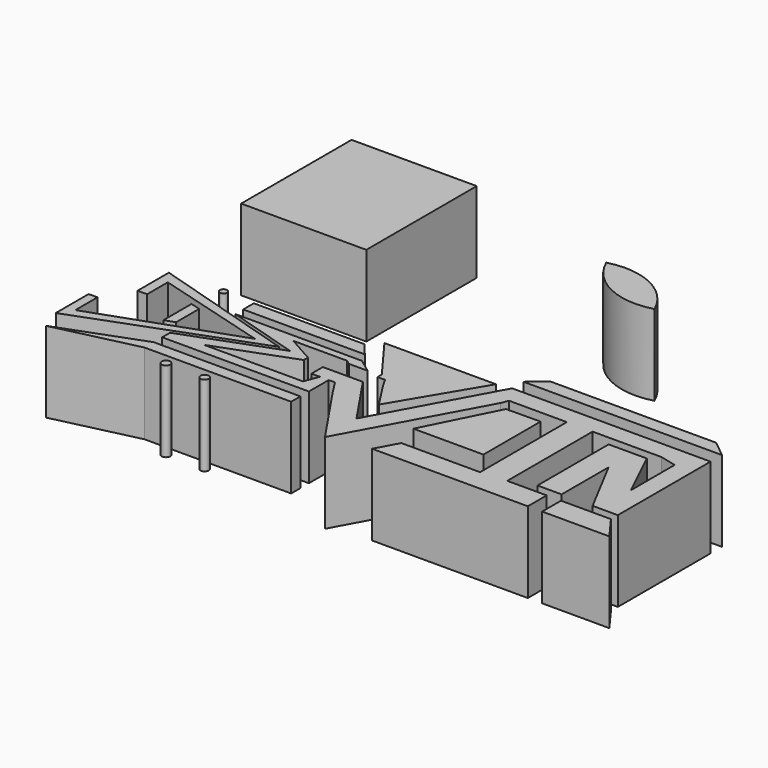
from build123d import *

# Parameters (mm, degrees)
F1_DEPTH = 25.4
F0_R     = 1.1458457214
F0_W     = 46.1219635762
F0_H     = 3.6322325468
F2_DEPTH = 25.4
F0_R_2   = 1.3357857731
F0_R_3   = 1.2844801698
F3_DEPTH = 25.4
F4_DEPTH = 25.4
F5_DEPTH = 25.4


# Not quite as in the source:
# - a feature names something its author has since deleted; it is built from what else it names


with BuildPart() as f1:
    # F0 (on Top) → F1 (new body)
    with BuildSketch(Plane.XY):
        Polygon((-6.457301788, -35.4142636061), (-52.2637851536, -21.4907061309), (-52.2637851536, -33.7999351323), (-49.2623485625, -33.7999351323), (-49.2623485625, -25.6701596081), (-13.7866064906, -35.7603244483), (-57.75090307, -51.3760596514), (-57.75090307, -42.6787286997), (-60.5372004211, -42.6787286997), (-60.5372004211, -55.5933304131), align=None)
    extrude(amount=F1_DEPTH)


with BuildPart() as f1b:
    # F0 (on Top) → F1, piece 2 (new body)
    with BuildSketch(Plane.XY):
        Polygon((-34.4110592502, -31.9099858361), (-37.5243715512, -31.024484012), (-37.5243715512, -42.071393411), (-34.4110592502, -40.9655719995), align=None)
    extrude(amount=F1_DEPTH)


with BuildPart() as f1c:
    # F0 (on Top) → F1, piece 3 (new body)
    with BuildSketch(Plane.XY):
        Polygon((-25.7907881661, -28.4884167007), (-3.0057569966, -35.4142636061), (-32.0811004348, -46.2632724339), (-32.0811004348, -49.3591018021), (14.0408631414, -49.3591018021), (14.0408631414, -41.5726949664), (16.0407461226, -41.5726949664), (18.8977234066, -46.0712859813), (32.2474647549, -65.7919248001), (54.5882796877, -24.7773277307), (55.4670058191, -22.503528744), (73.6564099789, -22.503528744), (73.6564099789, -56.5967746079), (48.895958811, -56.5967746079), (45.1729811572, -63.4316384583), (94.1314026713, -63.4316384583), (94.1314026713, -56.025378406), (81.7511752248, -56.025378406), (81.7511752248, -22.503528744), (103.4641936421, -22.503528744), (108.5540056229, -23.7593259662), (108.5540056229, -40.9735031426), (101.0794267058, -25.3448393196), (89.0748053789, -25.3448393196), (89.0748053789, -29.3086320162), (89.0748053789, -53.3178821206), (96.662633121, -53.3178821206), (96.662633121, -34.8579399288), (106.402233243, -53.3178821206), (114.3298149109, -53.3178821206), (114.3298149109, -16.8771834235), (103.4641936421, -16.8771834235), (51.9606553173, -16.8771834235), (48.8959625363, -22.503528744), (32.1416473914, -53.2620971716), (21.1833044887, -37.0741039515), (8.612611331, -37.0741039515), (8.612611331, -41.5726949664), (11.2791219726, -41.5726949664), (9.5649352297, -46.0712859813), (-21.4994866668, -46.0712859813), (2.6129609905, -37.0741039515), (2.6129609905, -35.4142636061), (-5.7674995624, -30.7306674425), (11.1563111566, -30.7306674425), (12.5171439722, -31.7410863936), (18.4215605259, -31.7410863936), (14.0408631414, -28.4884167007), align=None)
    extrude(amount=F1_DEPTH)


with BuildPart() as f1d:
    # F0 (on Top) → F1, piece 4 (new body)
    with BuildSketch(Plane.XY):
        Polygon((68.451821804, -26.3243597001), (57.6554350555, -26.4312550426), (46.4314706624, -48.7722866237), (68.451821804, -48.7722866237), align=None)
    extrude(amount=F1_DEPTH)


with BuildPart() as f1e:
    # F0 (on Top) → F1, piece 5 (new body)
    with BuildSketch(Plane.XY):
        Polygon((24.731811136, -32.8449457884), (26.2283403426, -35.4104228318), (31.7868739367, -44.0689101815), (47.5004203618, -17.6658723503), (12.4388998374, -17.6658723503), (22.3801247776, -31.1346296221), (22.3801247776, -32.8449457884), align=None)
    extrude(amount=F1_DEPTH)


with BuildPart() as f1f:
    # F0 (on Top) → F1, piece 6 (new body)
    with BuildSketch(Plane.XY):
        with Locations((-35.5569049716, -20.8727214485)):
            Circle(F0_R)
    extrude(amount=F1_DEPTH)


with BuildPart() as f2:
    # F0 (on Top) → F2 (new body)
    with BuildSketch(Plane.XY):
        with Locations((-9.0201186467, -54.49988693)):
            Rectangle(F0_W, F0_H)
        Polygon((-32.0811004348, -56.3160032034), (-32.0811004348, -52.6837706566), (-58.1316686189, -62.404131993), align=None)
    extrude(amount=F2_DEPTH)


with BuildPart() as f2b:
    # F0 (on Top) → F2, piece 2 (new body)
    with BuildSketch(Plane.XY):
        with Locations((-22.8066574782, -59.4273507595)):
            Circle(F0_R_2)
    extrude(amount=F2_DEPTH)


with BuildPart() as f2c:
    # F0 (on Top) → F2, piece 3 (new body)
    with BuildSketch(Plane.XY):
        with Locations((-10.6601277366, -59.4273507595)):
            Circle(F0_R_3)
    extrude(amount=F2_DEPTH)


with BuildPart() as f3:
    # F0 (on Top) → F3 (new body)
    with BuildSketch(Plane.XY):
        Polygon((56.9006577134, -8.172522299), (51.9606553173, -12.4101256952), (114.3298149109, -12.4101256952), (109.1644465923, -8.172522299), align=None)
    extrude(amount=F3_DEPTH)


with BuildPart() as f4:
    # F0 (on Top) → F4 (new body)
    with BuildSketch(Plane.XY):
        with BuildLine():
            ThreePointArc((-61.3443627954, 55.2970463574), (-59.4844908559, 59.7871744179), (-54.9943627954, 61.6470463574))
            Line((-54.9943627954, 61.6470463574), (-61.3443627954, 61.6470463574))
            Line((-61.3443627954, 61.6470463574), (-61.3443627954, 55.2970463574))
        make_face()
        with BuildLine():
            Line((-41.6697729379, 61.6470463574), (-54.9943627954, 61.6470463574))
            ThreePointArc((-54.9943627954, 61.6470463574), (-59.4844908559, 59.7871744179), (-61.3443627954, 55.2970463574))
            Line((-61.3443627954, 55.2970463574), (-61.3443627954, 39.9545514956))
            Line((-61.3443627954, 39.9545514956), (-41.6697729379, 39.9545514956))
            Line((-41.6697729379, 39.9545514956), (-41.6697729379, 61.6470463574))
        make_face()
        with BuildLine():
            Line((-28.3451830804, 61.6470463574), (-41.6697729379, 61.6470463574))
            Line((-41.6697729379, 61.6470463574), (-41.6697729379, 39.9545514956))
            Line((-41.6697729379, 39.9545514956), (-21.9951830804, 39.9545514956))
            Line((-21.9951830804, 39.9545514956), (-21.9951830804, 55.2970463574))
            ThreePointArc((-21.9951830804, 55.2970463574), (-23.8550550199, 59.7871744179), (-28.3451830804, 61.6470463574))
        make_face()
        with BuildLine():
            Line((-21.9951830804, 61.6470463574), (-28.3451830804, 61.6470463574))
            ThreePointArc((-28.3451830804, 61.6470463574), (-23.8550550199, 59.7871744179), (-21.9951830804, 55.2970463574))
            Line((-21.9951830804, 55.2970463574), (-21.9951830804, 61.6470463574))
        make_face()
        with BuildLine():
            Line((-21.9951830804, 39.9545514956), (-41.6697729379, 39.9545514956))
            Line((-41.6697729379, 39.9545514956), (-41.6697729379, 18.2620566338))
            Line((-41.6697729379, 18.2620566338), (-28.3451830804, 18.2620566338))
            ThreePointArc((-28.3451830804, 18.2620566338), (-23.8550550199, 20.1219285733), (-21.9951830804, 24.6120566338))
            Line((-21.9951830804, 24.6120566338), (-21.9951830804, 39.9545514956))
        make_face()
        with BuildLine():
            Line((-41.6697729379, 18.2620566338), (-41.6697729379, 39.9545514956))
            Line((-41.6697729379, 39.9545514956), (-61.3443627954, 39.9545514956))
            Line((-61.3443627954, 39.9545514956), (-61.3443627954, 24.6120566338))
            ThreePointArc((-61.3443627954, 24.6120566338), (-59.4844908559, 20.1219285733), (-54.9943627954, 18.2620566338))
            Line((-54.9943627954, 18.2620566338), (-41.6697729379, 18.2620566338))
        make_face()
        with BuildLine():
            ThreePointArc((-54.9943627954, 18.2620566338), (-59.4844908559, 20.1219285733), (-61.3443627954, 24.6120566338))
            Line((-61.3443627954, 24.6120566338), (-61.3443627954, 18.2620566338))
            Line((-61.3443627954, 18.2620566338), (-54.9943627954, 18.2620566338))
        make_face()
        with BuildLine():
            Line((-21.9951830804, 18.2620566338), (-21.9951830804, 24.6120566338))
            ThreePointArc((-21.9951830804, 24.6120566338), (-23.8550550199, 20.1219285733), (-28.3451830804, 18.2620566338))
            Line((-28.3451830804, 18.2620566338), (-21.9951830804, 18.2620566338))
        make_face()
    extrude(amount=F4_DEPTH)


with BuildPart() as f4b:
    # F0 (on Top) → F4, piece 2 (new body)
    with BuildSketch(Plane.XY):
        with BuildLine():
            ThreePointArc((28.2506924123, 49.7414022684), (38.3558151119, 39.1864963955), (52.9067942315, 37.849129796))
            ThreePointArc((52.9067942315, 37.849129796), (42.7947034208, 48.3895887704), (28.2506924123, 49.7414022684))
        make_face()
    extrude(amount=F4_DEPTH)


with BuildPart() as f4c:
    # F0 (on Top) → F4, piece 3 (new body)
    with BuildSketch(Plane.XY):
        Polygon((-6.457301788, -35.4142636061), (-52.2637851536, -21.4907061309), (-52.2637851536, -33.7999351323), (-49.2623485625, -33.7999351323), (-49.2623485625, -25.6701596081), (-13.7866064906, -35.7603244483), (-57.75090307, -51.3760596514), (-57.75090307, -42.6787286997), (-60.5372004211, -42.6787286997), (-60.5372004211, -55.5933304131), align=None)
    extrude(amount=F4_DEPTH)


with BuildPart() as f4d:
    # F0 (on Top) → F4, piece 4 (new body)
    with BuildSketch(Plane.XY):
        Polygon((-34.4110592502, -31.9099858361), (-37.5243715512, -31.024484012), (-37.5243715512, -42.071393411), (-34.4110592502, -40.9655719995), align=None)
    extrude(amount=F4_DEPTH)


with BuildPart() as f4e:
    # F0 (on Top) → F4, piece 5 (new body)
    with BuildSketch(Plane.XY):
        Polygon((-25.7907881661, -28.4884167007), (-3.0057569966, -35.4142636061), (-32.0811004348, -46.2632724339), (-32.0811004348, -49.3591018021), (14.0408631414, -49.3591018021), (14.0408631414, -41.5726949664), (16.0407461226, -41.5726949664), (18.8977234066, -46.0712859813), (32.2474647549, -65.7919248001), (54.5882796877, -24.7773277307), (55.4670058191, -22.503528744), (73.6564099789, -22.503528744), (73.6564099789, -56.5967746079), (48.895958811, -56.5967746079), (45.1729811572, -63.4316384583), (94.1314026713, -63.4316384583), (94.1314026713, -56.025378406), (81.7511752248, -56.025378406), (81.7511752248, -22.503528744), (103.4641936421, -22.503528744), (108.5540056229, -23.7593259662), (108.5540056229, -40.9735031426), (101.0794267058, -25.3448393196), (89.0748053789, -25.3448393196), (89.0748053789, -29.3086320162), (89.0748053789, -53.3178821206), (96.662633121, -53.3178821206), (96.662633121, -34.8579399288), (106.402233243, -53.3178821206), (114.3298149109, -53.3178821206), (114.3298149109, -16.8771834235), (103.4641936421, -16.8771834235), (51.9606553173, -16.8771834235), (48.8959625363, -22.503528744), (32.1416473914, -53.2620971716), (21.1833044887, -37.0741039515), (8.612611331, -37.0741039515), (8.612611331, -41.5726949664), (11.2791219726, -41.5726949664), (9.5649352297, -46.0712859813), (-21.4994866668, -46.0712859813), (2.6129609905, -37.0741039515), (2.6129609905, -35.4142636061), (-5.7674995624, -30.7306674425), (11.1563111566, -30.7306674425), (12.5171439722, -31.7410863936), (18.4215605259, -31.7410863936), (14.0408631414, -28.4884167007), align=None)
    extrude(amount=F4_DEPTH)


with BuildPart() as f4f:
    # F0 (on Top) → F4, piece 6 (new body)
    with BuildSketch(Plane.XY):
        Polygon((68.451821804, -26.3243597001), (57.6554350555, -26.4312550426), (46.4314706624, -48.7722866237), (68.451821804, -48.7722866237), align=None)
    extrude(amount=F4_DEPTH)


with BuildPart() as f4g:
    # F0 (on Top) → F4, piece 7 (new body)
    with BuildSketch(Plane.XY):
        Polygon((24.731811136, -32.8449457884), (26.2283403426, -35.4104228318), (31.7868739367, -44.0689101815), (47.5004203618, -17.6658723503), (12.4388998374, -17.6658723503), (22.3801247776, -31.1346296221), (22.3801247776, -32.8449457884), align=None)
    extrude(amount=F4_DEPTH)


with BuildPart() as f4h:
    # F0 (on Top) → F4, piece 8 (new body)
    with BuildSketch(Plane.XY):
        with Locations((-35.5569049716, -20.8727214485)):
            Circle(F0_R)
    extrude(amount=F4_DEPTH)


with BuildPart() as f4i:
    # F0 (on Top) → F4, piece 9 (new body)
    with BuildSketch(Plane.XY):
        with Locations((-9.0201186467, -54.49988693)):
            Rectangle(F0_W, F0_H)
        Polygon((-32.0811004348, -56.3160032034), (-32.0811004348, -52.6837706566), (-58.1316686189, -62.404131993), align=None)
    extrude(amount=F4_DEPTH)


with BuildPart() as f4j:
    # F0 (on Top) → F4, piece 10 (new body)
    with BuildSketch(Plane.XY):
        with Locations((-22.8066574782, -59.4273507595)):
            Circle(F0_R_2)
    extrude(amount=F4_DEPTH)


with BuildPart() as f4k:
    # F0 (on Top) → F4, piece 11 (new body)
    with BuildSketch(Plane.XY):
        with Locations((-10.6601277366, -59.4273507595)):
            Circle(F0_R_3)
    extrude(amount=F4_DEPTH)


with BuildPart() as f4l:
    # F0 (on Top) → F4, piece 12 (new body)
    with BuildSketch(Plane.XY):
        Polygon((56.9006577134, -8.172522299), (51.9606553173, -12.4101256952), (114.3298149109, -12.4101256952), (109.1644465923, -8.172522299), align=None)
    extrude(amount=F4_DEPTH)


with BuildPart() as f4m:
    # F0 (on Top) → F4, piece 13 (new body)
    with BuildSketch(Plane.XY):
        Polygon((98.6332297325, -56.025378406), (98.6332297325, -63.4316384583), (119.7509765625, -63.4316384583), (114.3298149109, -56.025378406), align=None)
    extrude(amount=F4_DEPTH)


with BuildPart() as f4n:
    # F0 (on Top) → F4, piece 14 (new body)
    with BuildSketch(Plane.XY):
        Polygon((-25.7907881661, -21.1860779673), (-25.7907881661, -25.376310572), (12.4349221587, -25.376310572), (9.0065514669, -21.1860779673), align=None)
    extrude(amount=F4_DEPTH)


with BuildPart() as f5:
    # F0 (on Top) → F5 (new body)
    with BuildSketch(Plane.XY):
        with BuildLine():
            ThreePointArc((-61.3443627954, 55.2970463574), (-59.4844908559, 59.7871744179), (-54.9943627954, 61.6470463574))
            Line((-54.9943627954, 61.6470463574), (-61.3443627954, 61.6470463574))
            Line((-61.3443627954, 61.6470463574), (-61.3443627954, 55.2970463574))
        make_face()
        with BuildLine():
            Line((-41.6697729379, 61.6470463574), (-54.9943627954, 61.6470463574))
            ThreePointArc((-54.9943627954, 61.6470463574), (-59.4844908559, 59.7871744179), (-61.3443627954, 55.2970463574))
            Line((-61.3443627954, 55.2970463574), (-61.3443627954, 39.9545514956))
            Line((-61.3443627954, 39.9545514956), (-41.6697729379, 39.9545514956))
            Line((-41.6697729379, 39.9545514956), (-41.6697729379, 61.6470463574))
        make_face()
        with BuildLine():
            Line((-28.3451830804, 61.6470463574), (-41.6697729379, 61.6470463574))
            Line((-41.6697729379, 61.6470463574), (-41.6697729379, 39.9545514956))
            Line((-41.6697729379, 39.9545514956), (-21.9951830804, 39.9545514956))
            Line((-21.9951830804, 39.9545514956), (-21.9951830804, 55.2970463574))
            ThreePointArc((-21.9951830804, 55.2970463574), (-23.8550550199, 59.7871744179), (-28.3451830804, 61.6470463574))
        make_face()
        with BuildLine():
            Line((-21.9951830804, 61.6470463574), (-28.3451830804, 61.6470463574))
            ThreePointArc((-28.3451830804, 61.6470463574), (-23.8550550199, 59.7871744179), (-21.9951830804, 55.2970463574))
            Line((-21.9951830804, 55.2970463574), (-21.9951830804, 61.6470463574))
        make_face()
        with BuildLine():
            Line((-21.9951830804, 39.9545514956), (-41.6697729379, 39.9545514956))
            Line((-41.6697729379, 39.9545514956), (-41.6697729379, 18.2620566338))
            Line((-41.6697729379, 18.2620566338), (-28.3451830804, 18.2620566338))
            ThreePointArc((-28.3451830804, 18.2620566338), (-23.8550550199, 20.1219285733), (-21.9951830804, 24.6120566338))
            Line((-21.9951830804, 24.6120566338), (-21.9951830804, 39.9545514956))
        make_face()
        with BuildLine():
            Line((-41.6697729379, 18.2620566338), (-41.6697729379, 39.9545514956))
            Line((-41.6697729379, 39.9545514956), (-61.3443627954, 39.9545514956))
            Line((-61.3443627954, 39.9545514956), (-61.3443627954, 24.6120566338))
            ThreePointArc((-61.3443627954, 24.6120566338), (-59.4844908559, 20.1219285733), (-54.9943627954, 18.2620566338))
            Line((-54.9943627954, 18.2620566338), (-41.6697729379, 18.2620566338))
        make_face()
        with BuildLine():
            ThreePointArc((-54.9943627954, 18.2620566338), (-59.4844908559, 20.1219285733), (-61.3443627954, 24.6120566338))
            Line((-61.3443627954, 24.6120566338), (-61.3443627954, 18.2620566338))
            Line((-61.3443627954, 18.2620566338), (-54.9943627954, 18.2620566338))
        make_face()
        with BuildLine():
            Line((-21.9951830804, 18.2620566338), (-21.9951830804, 24.6120566338))
            ThreePointArc((-21.9951830804, 24.6120566338), (-23.8550550199, 20.1219285733), (-28.3451830804, 18.2620566338))
            Line((-28.3451830804, 18.2620566338), (-21.9951830804, 18.2620566338))
        make_face()
    extrude(amount=F5_DEPTH)


with BuildPart() as f5b:
    # F0 (on Top) → F5, piece 2 (new body)
    with BuildSketch(Plane.XY):
        with BuildLine():
            ThreePointArc((28.2506924123, 49.7414022684), (38.3558151119, 39.1864963955), (52.9067942315, 37.849129796))
            ThreePointArc((52.9067942315, 37.849129796), (42.7947034208, 48.3895887704), (28.2506924123, 49.7414022684))
        make_face()
    extrude(amount=F5_DEPTH)


with BuildPart() as f5c:
    # F0 (on Top) → F5, piece 3 (new body)
    with BuildSketch(Plane.XY):
        Polygon((-6.457301788, -35.4142636061), (-52.2637851536, -21.4907061309), (-52.2637851536, -33.7999351323), (-49.2623485625, -33.7999351323), (-49.2623485625, -25.6701596081), (-13.7866064906, -35.7603244483), (-57.75090307, -51.3760596514), (-57.75090307, -42.6787286997), (-60.5372004211, -42.6787286997), (-60.5372004211, -55.5933304131), align=None)
    extrude(amount=F5_DEPTH)


with BuildPart() as f5d:
    # F0 (on Top) → F5, piece 4 (new body)
    with BuildSketch(Plane.XY):
        Polygon((-34.4110592502, -31.9099858361), (-37.5243715512, -31.024484012), (-37.5243715512, -42.071393411), (-34.4110592502, -40.9655719995), align=None)
    extrude(amount=F5_DEPTH)


with BuildPart() as f5e:
    # F0 (on Top) → F5, piece 5 (new body)
    with BuildSketch(Plane.XY):
        Polygon((-25.7907881661, -28.4884167007), (-3.0057569966, -35.4142636061), (-32.0811004348, -46.2632724339), (-32.0811004348, -49.3591018021), (14.0408631414, -49.3591018021), (14.0408631414, -41.5726949664), (16.0407461226, -41.5726949664), (18.8977234066, -46.0712859813), (32.2474647549, -65.7919248001), (54.5882796877, -24.7773277307), (55.4670058191, -22.503528744), (73.6564099789, -22.503528744), (73.6564099789, -56.5967746079), (48.895958811, -56.5967746079), (45.1729811572, -63.4316384583), (94.1314026713, -63.4316384583), (94.1314026713, -56.025378406), (81.7511752248, -56.025378406), (81.7511752248, -22.503528744), (103.4641936421, -22.503528744), (108.5540056229, -23.7593259662), (108.5540056229, -40.9735031426), (101.0794267058, -25.3448393196), (89.0748053789, -25.3448393196), (89.0748053789, -29.3086320162), (89.0748053789, -53.3178821206), (96.662633121, -53.3178821206), (96.662633121, -34.8579399288), (106.402233243, -53.3178821206), (114.3298149109, -53.3178821206), (114.3298149109, -16.8771834235), (103.4641936421, -16.8771834235), (51.9606553173, -16.8771834235), (48.8959625363, -22.503528744), (32.1416473914, -53.2620971716), (21.1833044887, -37.0741039515), (8.612611331, -37.0741039515), (8.612611331, -41.5726949664), (11.2791219726, -41.5726949664), (9.5649352297, -46.0712859813), (-21.4994866668, -46.0712859813), (2.6129609905, -37.0741039515), (2.6129609905, -35.4142636061), (-5.7674995624, -30.7306674425), (11.1563111566, -30.7306674425), (12.5171439722, -31.7410863936), (18.4215605259, -31.7410863936), (14.0408631414, -28.4884167007), align=None)
    extrude(amount=F5_DEPTH)


with BuildPart() as f5f:
    # F0 (on Top) → F5, piece 6 (new body)
    with BuildSketch(Plane.XY):
        Polygon((68.451821804, -26.3243597001), (57.6554350555, -26.4312550426), (46.4314706624, -48.7722866237), (68.451821804, -48.7722866237), align=None)
    extrude(amount=F5_DEPTH)


with BuildPart() as f5g:
    # F0 (on Top) → F5, piece 7 (new body)
    with BuildSketch(Plane.XY):
        Polygon((24.731811136, -32.8449457884), (26.2283403426, -35.4104228318), (31.7868739367, -44.0689101815), (47.5004203618, -17.6658723503), (12.4388998374, -17.6658723503), (22.3801247776, -31.1346296221), (22.3801247776, -32.8449457884), align=None)
    extrude(amount=F5_DEPTH)


with BuildPart() as f5h:
    # F0 (on Top) → F5, piece 8 (new body)
    with BuildSketch(Plane.XY):
        with Locations((-35.5569049716, -20.8727214485)):
            Circle(F0_R)
    extrude(amount=F5_DEPTH)


with BuildPart() as f5i:
    # F0 (on Top) → F5, piece 9 (new body)
    with BuildSketch(Plane.XY):
        with Locations((-9.0201186467, -54.49988693)):
            Rectangle(F0_W, F0_H)
        Polygon((-32.0811004348, -56.3160032034), (-32.0811004348, -52.6837706566), (-58.1316686189, -62.404131993), align=None)
    extrude(amount=F5_DEPTH)


with BuildPart() as f5j:
    # F0 (on Top) → F5, piece 10 (new body)
    with BuildSketch(Plane.XY):
        with Locations((-22.8066574782, -59.4273507595)):
            Circle(F0_R_2)
    extrude(amount=F5_DEPTH)


with BuildPart() as f5k:
    # F0 (on Top) → F5, piece 11 (new body)
    with BuildSketch(Plane.XY):
        with Locations((-10.6601277366, -59.4273507595)):
            Circle(F0_R_3)
    extrude(amount=F5_DEPTH)


with BuildPart() as f5l:
    # F0 (on Top) → F5, piece 12 (new body)
    with BuildSketch(Plane.XY):
        Polygon((56.9006577134, -8.172522299), (51.9606553173, -12.4101256952), (114.3298149109, -12.4101256952), (109.1644465923, -8.172522299), align=None)
    extrude(amount=F5_DEPTH)


with BuildPart() as f5m:
    # F0 (on Top) → F5, piece 13 (new body)
    with BuildSketch(Plane.XY):
        Polygon((98.6332297325, -56.025378406), (98.6332297325, -63.4316384583), (119.7509765625, -63.4316384583), (114.3298149109, -56.025378406), align=None)
    extrude(amount=F5_DEPTH)


with BuildPart() as f5n:
    # F0 (on Top) → F5, piece 14 (new body)
    with BuildSketch(Plane.XY):
        Polygon((-25.7907881661, -21.1860779673), (-25.7907881661, -25.376310572), (12.4349221587, -25.376310572), (9.0065514669, -21.1860779673), align=None)
    extrude(amount=F5_DEPTH)


solid = Compound([f1.part, f1b.part, f1c.part, f1d.part, f1e.part, f1f.part, f2.part, f2b.part, f2c.part, f3.part, f4.part, f4b.part, f4c.part, f4d.part, f4e.part, f4f.part, f4g.part, f4h.part, f4i.part, f4j.part, f4k.part, f4l.part, f4m.part, f4n.part, f5.part, f5b.part, f5c.part, f5d.part, f5e.part, f5f.part, f5g.part, f5h.part, f5i.part, f5j.part, f5k.part, f5l.part, f5m.part, f5n.part])
